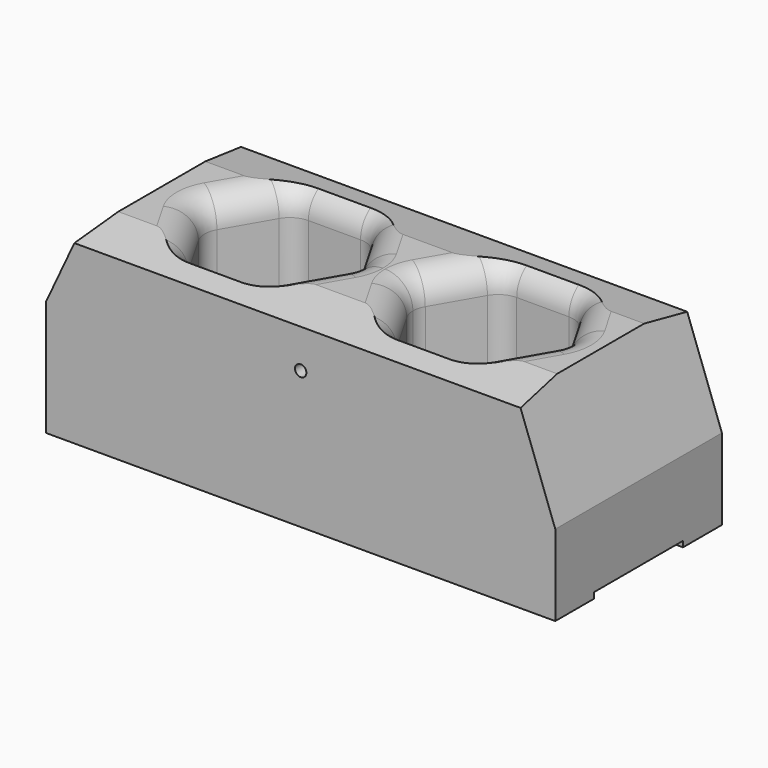
from build123d import *

# Parameters (mm, degrees)
F0_W      = 220
F0_H      = 90
F1_DEPTH  = 80
F3_DEPTH  = 80.001
F4_R      = 12
F6_DEPTH  = 90
F8_DEPTH  = 220.001
F9_R      = 2.465
F10_DEPTH = 23.18
F11_R     = 2.465
F12_DEPTH = 23.5
F13_R     = 2.43
F14_DEPTH = 23
F13_R_2   = 3.56
F15_DEPTH = 25.5


# Not quite as in the source:
# - a feature names something its author has since deleted; it is built from what else it names


with BuildPart() as f1:
    # F0 (on Top) → F1 (new body)
    with BuildSketch(Plane.XY):
        Rectangle(F0_W, F0_H)
    extrude(amount=F1_DEPTH)

    # F2 (on face) → F3 (cut, through all)
    with BuildSketch(Plane(origin=(0, 0, 0), x_dir=(1, 0, 0), z_dir=(0, 0, -1))):
        with BuildLine():
            ThreePointArc((-13.8230854638, -5), (-12.8240812387, -2.588190451), (-12.4833395016, 0))
            Line((-12.4833395016, 0), (-45, 0))
            Line((-45, 0), (-45, 29.5))
            Line((-45, 29.5), (-56.2583302492, 29.5))
            ThreePointArc((-56.2583302492, 29.5), (-61.2583302492, 28.1602540378), (-64.918584287, 24.5))
            Line((-64.918584287, 24.5), (-76.1769145362, 5))
            ThreePointArc((-76.1769145362, 5), (-77.5166604984, 0), (-76.1769145362, -5))
            Line((-76.1769145362, -5), (-64.918584287, -24.5))
            ThreePointArc((-64.918584287, -24.5), (-61.2583302492, -28.1602540378), (-56.2583302492, -29.5))
            Line((-56.2583302492, -29.5), (-33.7416697508, -29.5))
            ThreePointArc((-33.7416697508, -29.5), (-28.7416697508, -28.1602540378), (-25.081415713, -24.5))
            Line((-25.081415713, -24.5), (-13.8230854638, -5))
        make_face()
        with BuildLine():
            Line((-45, 0), (-12.4833395016, 0))
            ThreePointArc((-12.4833395016, 0), (-12.8240812387, 2.588190451), (-13.8230854638, 5))
            Line((-13.8230854638, 5), (-25.081415713, 24.5))
            ThreePointArc((-25.081415713, 24.5), (-28.7416697508, 28.1602540378), (-33.7416697508, 29.5))
            Line((-33.7416697508, 29.5), (-45, 29.5))
            Line((-45, 29.5), (-45, 0))
        make_face()
        with BuildLine():
            ThreePointArc((13.8230854638, 5), (12.8240812387, 2.588190451), (12.4833395016, 0))
            Line((12.4833395016, 0), (45, 0))
            Line((45, 0), (45, 29.5))
            Line((45, 29.5), (33.7416697508, 29.5))
            ThreePointArc((33.7416697508, 29.5), (28.7416697508, 28.1602540378), (25.081415713, 24.5))
            Line((25.081415713, 24.5), (13.8230854638, 5))
        make_face()
        with BuildLine():
            Line((45, 0), (12.4833395016, 0))
            ThreePointArc((12.4833395016, 0), (12.8240812387, -2.588190451), (13.8230854638, -5))
            Line((13.8230854638, -5), (25.081415713, -24.5))
            ThreePointArc((25.081415713, -24.5), (28.7416697508, -28.1602540378), (33.7416697508, -29.5))
            Line((33.7416697508, -29.5), (56.2583302492, -29.5))
            ThreePointArc((56.2583302492, -29.5), (61.2583302492, -28.1602540378), (64.918584287, -24.5))
            Line((64.918584287, -24.5), (76.1769145362, -5))
            ThreePointArc((76.1769145362, -5), (77.5166604984, 0), (76.1769145362, 5))
            Line((76.1769145362, 5), (64.918584287, 24.5))
            ThreePointArc((64.918584287, 24.5), (61.2583302492, 28.1602540378), (56.2583302492, 29.5))
            Line((56.2583302492, 29.5), (45, 29.5))
            Line((45, 29.5), (45, 0))
        make_face()
    extrude(amount=-F3_DEPTH, mode=Mode.SUBTRACT)

    # F4
    f4_edges = [f1.edges().sort_by_distance(p)[0] for p in [
        (-45, 29.5, 80),
        (45, 29.5, 80),
    ]]
    fillet(f4_edges, radius=F4_R)

    # F5 (on face) → F6 (cut)
    with BuildSketch(Plane.XZ.offset(45)):
        Polygon((-110, 80), (-110, 50), (-96.0107702554, 80), align=None)
        Polygon((110, 80), (93.621339458, 80), (110, 35), align=None)
    extrude(amount=-F6_DEPTH, mode=Mode.SUBTRACT)

    # F7 (on face) → F8 (cut, through all)
    with BuildSketch(Plane(origin=(-110, 0, 0), x_dir=(0, -1, 0), z_dir=(-1, 0, 0))):
        Polygon((-23.5, 80), (-45, 80), (-45, 76.2089699148), align=None)
        Polygon((23.5, 80), (45, 76.2089699148), (45, 78.1686380506), (45, 80), align=None)
        Polygon((-24, 0), (0, 0), (24, 0), (24, 2.5), (-24, 2.5), align=None)
    extrude(amount=-F8_DEPTH, mode=Mode.SUBTRACT)

    # F9 (on face) → F10 (cut)
    with BuildSketch(Plane(origin=(-110, 0, 0), x_dir=(0, -1, 0), z_dir=(-1, 0, 0))):
        with Locations((0, 47)):
            Circle(F9_R)
    extrude(amount=-F10_DEPTH, mode=Mode.SUBTRACT)

    # F11 (on face) → F12 (cut)
    with BuildSketch(Plane.XZ.offset(45)):
        with Locations((0, 59.465)):
            Circle(F11_R)
    extrude(amount=-F12_DEPTH, mode=Mode.SUBTRACT)

    # F13 (on face) → F14 (cut)
    with BuildSketch(Plane(origin=(0, 0, 0), x_dir=(1, 0, 0), z_dir=(0, 0, -1))):
        with Locations((-91.5, 30)):
            Circle(F13_R)
        with Locations((91.5, 30)):
            Circle(F13_R)
        with Locations((91.5, -30)):
            Circle(F13_R)
        with Locations((-91.5, -30)):
            Circle(F13_R)
    extrude(amount=-F14_DEPTH, mode=Mode.SUBTRACT)

    # F13 (on face) → F15 (cut)
    with BuildSketch(Plane(origin=(0, 0, 0), x_dir=(1, 0, 0), z_dir=(0, 0, -1))):
        with Locations((-96.5, 12.9)):
            Circle(F13_R_2)
        with Locations((-96.5, -12.9)):
            Circle(F13_R_2)
        with Locations((96.5, -12.9)):
            Circle(F13_R_2)
        with Locations((96.5, 12.9)):
            Circle(F13_R_2)
    extrude(amount=-F15_DEPTH, mode=Mode.SUBTRACT)


solid = f1.part
